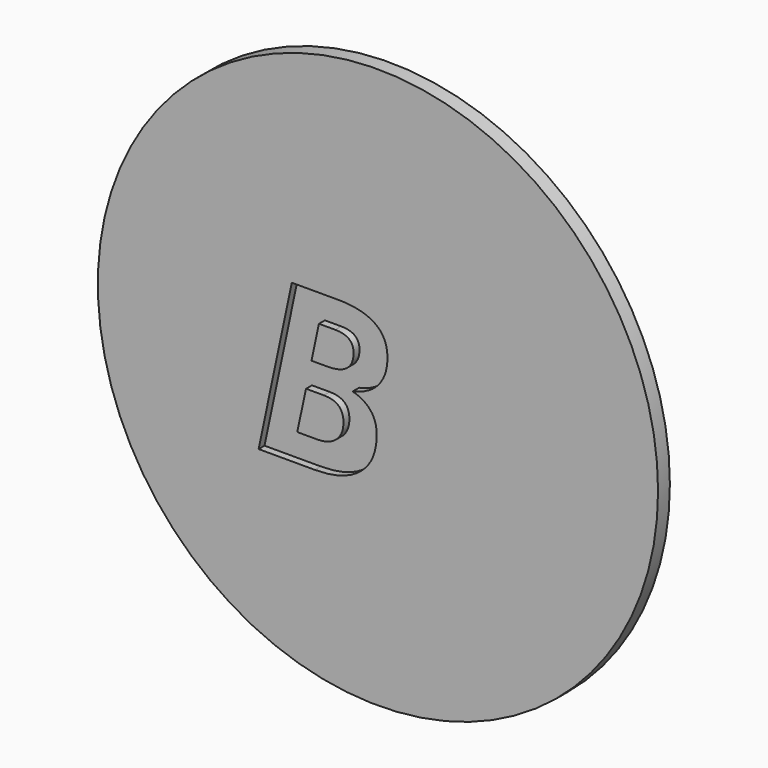
from build123d import *

# Parameters (mm, degrees)
F0_R         = 37.8965637932
F1_DEPTH     = 2
F2_TEXT_SIZE = 29.8077628637
F3_DEPTH     = 1


# Not quite as in the source:
# - Text() gives the source's letters only with a copy of the font that has no kerning and outlines rounded to 1/6400 em; it was checked with that copy


with BuildPart() as f1:
    # F0 (on Front) → F1 (new body)
    with BuildSketch(Plane.XZ):
        with Locations((-39.4791513681, 36.8948057294)):
            Circle(F0_R)
    extrude(amount=F1_DEPTH)

    # F2 (on face) → F3 (cut)
    with BuildSketch(Plane.XZ.offset(2)):
        with Locations((-56.3987791538, 24.2961477488)):
            Text('B', F2_TEXT_SIZE, font='Open Sans', font_style=FontStyle.BOLDITALIC, text_align=(TextAlign.LEFT, TextAlign.BOTTOM))
    extrude(amount=-F3_DEPTH, mode=Mode.SUBTRACT)


solid = f1.part
